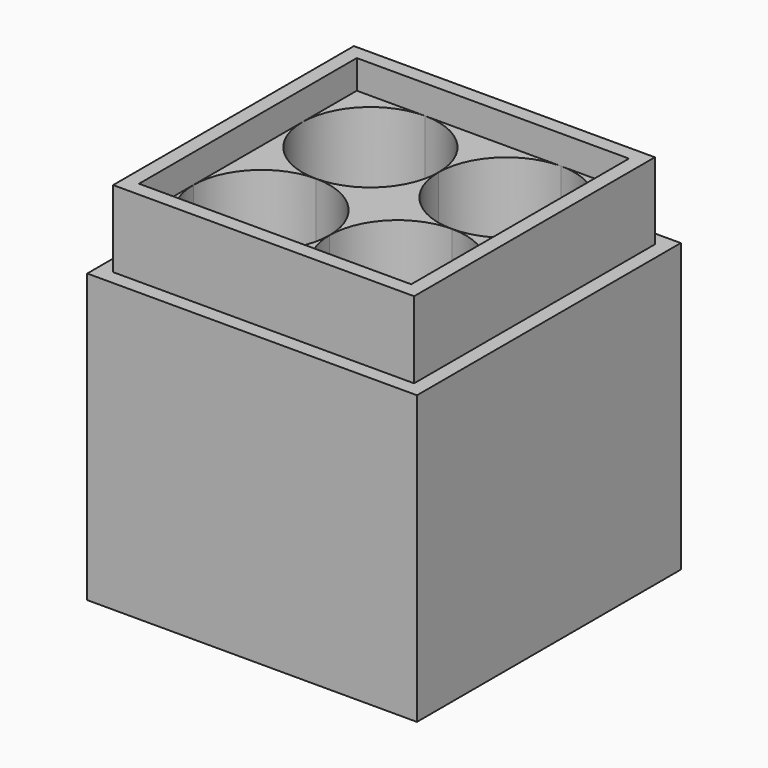
from build123d import *

# Parameters (mm, degrees)
F0_W     = 31.4
F0_H     = 31.4
F1_DEPTH = 38
F0_W_2   = 34.4
F0_H_2   = 34.4
F2_DEPTH = 30
F3_DEPTH = 35
F4_DEPTH = 3


with BuildPart() as f1:
    # F0 (on Top) → F1 (new body)
    with BuildSketch(Plane.XY):
        Rectangle(F0_W, F0_H)
        Polygon((7.1, 14.2), (14.2, 14.2), (14.2, 7.1), (14.2, -7.1), (14.2, -14.2), (7.1, -14.2), (-7.1000000056, -14.2), (-14.2, -14.2), (-14.2, -7.1), (-14.2, 7.1), (-14.2, 14.2), (-7.0999999722, 14.2), align=None, mode=Mode.SUBTRACT)
    extrude(amount=F1_DEPTH)

    # F0 (on Top) → F2 (join)
    with BuildSketch(Plane.XY):
        Rectangle(F0_W_2, F0_H_2)
        Rectangle(F0_W, F0_H, mode=Mode.SUBTRACT)
    extrude(amount=F2_DEPTH)

    # F0 (on Top) → F3, piece 2 (join)
    with BuildSketch(Plane.XY):
        with BuildLine():
            ThreePointArc((-14.2, 7.1), (-12.1204581366, 12.1204581563), (-7.0999999722, 14.2))
            Line((-7.0999999722, 14.2), (-14.2, 14.2))
            Line((-14.2, 14.2), (-14.2, 7.1))
        make_face()
        with BuildLine():
            ThreePointArc((0, 7.1), (2.0795418536, 12.1204581464), (7.1, 14.2))
            Line((7.1, 14.2), (-7.0999999722, 14.2))
            ThreePointArc((-7.0999999722, 14.2), (-2.0795418437, 12.1204581366), (0, 7.1))
        make_face()
        with BuildLine():
            Line((14.2, 7.1), (14.2, 14.2))
            Line((14.2, 14.2), (7.1, 14.2))
            ThreePointArc((7.1, 14.2), (12.1204581464, 12.1204581464), (14.2, 7.1))
        make_face()
        with BuildLine():
            Line((14.2, -7.1), (14.2, 7.1))
            ThreePointArc((14.2, 7.1), (12.1204581464, 2.0795418536), (7.1, 0))
            ThreePointArc((7.1, 0), (12.1204581464, -2.0795418536), (14.2, -7.1))
        make_face()
        with BuildLine():
            ThreePointArc((-7.1, 0), (-12.1204581464, 2.0795418536), (-14.2, 7.1))
            Line((-14.2, 7.1), (-14.2, -7.1))
            ThreePointArc((-14.2, -7.1), (-12.1204581464, -2.0795418536), (-7.1, 0))
        make_face()
        with BuildLine():
            ThreePointArc((-7.1000000056, -14.2), (-12.1204581484, -12.1204581444), (-14.2, -7.1))
            Line((-14.2, -7.1), (-14.2, -14.2))
            Line((-14.2, -14.2), (-7.1000000056, -14.2))
        make_face()
        with BuildLine():
            Line((-7.1000000056, -14.2), (7.1, -14.2))
            ThreePointArc((7.1, -14.2), (2.0795418536, -12.1204581464), (0, -7.1))
            ThreePointArc((0, -7.1), (-2.0795418556, -12.1204581484), (-7.1000000056, -14.2))
        make_face()
        with BuildLine():
            Line((14.2, -14.2), (14.2, -7.1))
            ThreePointArc((14.2, -7.1), (12.1204581464, -12.1204581464), (7.1, -14.2))
            Line((7.1, -14.2), (14.2, -14.2))
        make_face()
    extrude(amount=F3_DEPTH)

    # F0 (on Top) → F4 (join)
    with BuildSketch(Plane.XY):
        with BuildLine():
            Line((-7.1, -7.1), (-7.1, 0))
            ThreePointArc((-7.1, 0), (-12.1204581464, -2.0795418536), (-14.2, -7.1))
            ThreePointArc((-14.2, -7.1), (-12.1204581484, -12.1204581444), (-7.1000000056, -14.2))
            ThreePointArc((-7.1000000056, -14.2), (-2.0795418556, -12.1204581484), (0, -7.1))
            Line((0, -7.1), (-7.1, -7.1))
        make_face()
        with BuildLine():
            ThreePointArc((0, 7.1), (-2.0795418437, 12.1204581366), (-7.0999999722, 14.2))
            ThreePointArc((-7.0999999722, 14.2), (-12.1204581366, 12.1204581563), (-14.2, 7.1))
            ThreePointArc((-14.2, 7.1), (-12.1204581464, 2.0795418536), (-7.1, 0))
            Line((-7.1, 0), (-7.1, 7.1))
            Line((-7.1, 7.1), (0, 7.1))
        make_face()
        with BuildLine():
            ThreePointArc((0, -7.1), (-2.0795418536, -2.0795418536), (-7.1, 0))
            Line((-7.1, 0), (-7.1, -7.1))
            Line((-7.1, -7.1), (0, -7.1))
        make_face()
        with BuildLine():
            ThreePointArc((-7.1, 0), (-2.0795418536, 2.0795418536), (0, 7.1))
            Line((0, 7.1), (-7.1, 7.1))
            Line((-7.1, 7.1), (-7.1, 0))
        make_face()
        with BuildLine():
            ThreePointArc((7.1, -14.2), (12.1204581464, -12.1204581464), (14.2, -7.1))
            ThreePointArc((14.2, -7.1), (12.1204581464, -2.0795418536), (7.1, 0))
            Line((7.1, 0), (7.1, -7.1))
            Line((7.1, -7.1), (0, -7.1))
            ThreePointArc((0, -7.1), (2.0795418536, -12.1204581464), (7.1, -14.2))
        make_face()
        with BuildLine():
            Line((7.1, -7.1), (7.1, 0))
            ThreePointArc((7.1, 0), (2.0795418536, -2.0795418536), (0, -7.1))
            Line((0, -7.1), (7.1, -7.1))
        make_face()
        with BuildLine():
            ThreePointArc((14.2, 7.1), (12.1204581464, 12.1204581464), (7.1, 14.2))
            ThreePointArc((7.1, 14.2), (2.0795418536, 12.1204581464), (0, 7.1))
            Line((0, 7.1), (7.1, 7.1))
            Line((7.1, 7.1), (7.1, 0))
            ThreePointArc((7.1, 0), (12.1204581464, 2.0795418536), (14.2, 7.1))
        make_face()
        with BuildLine():
            Line((7.1, 7.1), (0, 7.1))
            ThreePointArc((0, 7.1), (2.0795418536, 2.0795418536), (7.1, 0))
            Line((7.1, 0), (7.1, 7.1))
        make_face()
    extrude(amount=F4_DEPTH)


with BuildPart() as f3:
    # F0 (on Top) → F3 (new body)
    with BuildSketch(Plane.XY):
        with BuildLine():
            ThreePointArc((7.1, 0), (2.0795418536, 2.0795418536), (0, 7.1))
            Line((0, 7.1), (0, 0))
            Line((0, 0), (7.1, 0))
        make_face()
        with BuildLine():
            Line((0, 0), (0, 7.1))
            ThreePointArc((0, 7.1), (-2.0795418536, 2.0795418536), (-7.1, 0))
            Line((-7.1, 0), (0, 0))
        make_face()
        with BuildLine():
            Line((0, -7.1), (0, 0))
            Line((0, 0), (-7.1, 0))
            ThreePointArc((-7.1, 0), (-2.0795418536, -2.0795418536), (0, -7.1))
        make_face()
        with BuildLine():
            ThreePointArc((0, -7.1), (2.0795418536, -2.0795418536), (7.1, 0))
            Line((7.1, 0), (0, 0))
            Line((0, 0), (0, -7.1))
        make_face()
    extrude(amount=F3_DEPTH)


solid = Compound([f1.part, f3.part])
